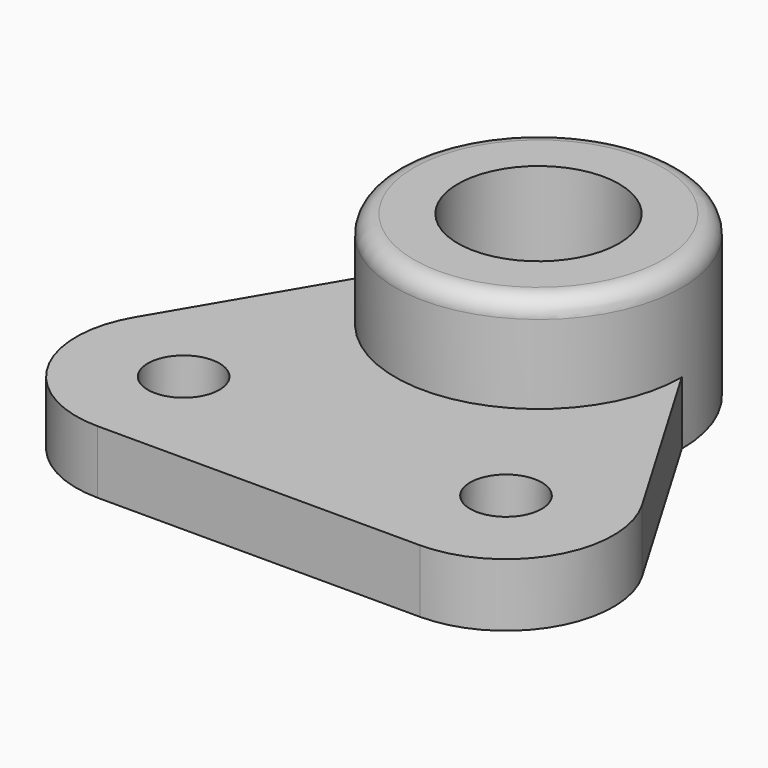
from build123d import *

# Parameters (mm, degrees)
F0_R     = 14.2875
F1_DEPTH = 28.448
F0_R_2   = 6.35
F2_DEPTH = 11.176
F3_R     = 3.302


with BuildPart() as f1:
    # F0 (on Top) → F1 (new body)
    with BuildSketch(Plane.XY):
        with BuildLine():
            ThreePointArc((25.4, 61.976), (0, 87.376), (-25.4, 61.976))
            ThreePointArc((-25.4, 61.976), (0, 36.576), (25.4, 61.976))
        make_face()
        with Locations((0, 61.976)):
            Circle(F0_R, mode=Mode.SUBTRACT)
    extrude(amount=F1_DEPTH)

    # F0 (on Top) → F2 (join)
    with BuildSketch(Plane.XY):
        with BuildLine():
            Line((-28.575, 0), (0, 0))
            Line((0, 0), (28.575, 0))
            ThreePointArc((28.575, 0), (45.1140748574, 9.5968786709), (44.989265753, 28.7182149226))
            Line((44.989265753, 28.7182149226), (25.4, 61.976))
            ThreePointArc((25.4, 61.976), (0, 36.576), (-25.4, 61.976))
            Line((-25.4, 61.976), (-44.989265753, 28.7182149226))
            ThreePointArc((-44.989265753, 28.7182149226), (-45.1140748574, 9.5968786709), (-28.575, 0))
        make_face()
        with Locations((-28.575, 19.05)):
            Circle(F0_R_2, mode=Mode.SUBTRACT)
        with Locations((28.575, 19.05)):
            Circle(F0_R_2, mode=Mode.SUBTRACT)
    extrude(amount=F2_DEPTH)

    # F3
    f3_edges = [f1.edges().sort_by_distance(p)[0] for p in [
        (25.4, 61.976, 28.448),
    ]]
    fillet(f3_edges, radius=F3_R)


solid = f1.part
